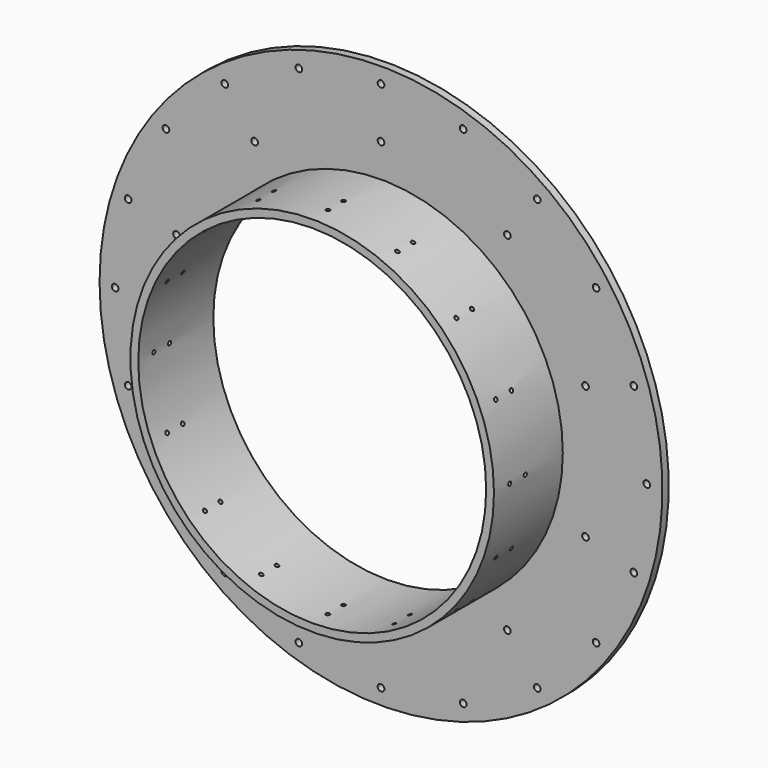
from build123d import *

# Parameters (mm, degrees)
F0_R            = 232.5
F0_R_2          = 222.5
F1_DEPTH        = 60
F2_R            = 360
F2_R_2          = 232.5
F3_DEPTH        = 10
F5_D            = 8.5
F5_DEPTH        = 30
F5_TIP          = 2.5536576309
F5_COPIES_COUNT = 10
F6_R            = 2.5
F7_DEPTH        = 300
F7_COPIES_COUNT = 16
F9_D            = 8.5
F9_DEPTH        = 22.1
F9_TIP          = 2.5536576309
F9_COPIES_COUNT = 20


# Not quite as in the source:
# - a pattern or mirror of a feature is missing from the dataset's text; its kind, count and spacing are read off the source's solid


with BuildPart() as f1:
    # F0 (on Front) → F1 (new body, symmetric)
    with BuildSketch(Plane.XZ):
        Circle(F0_R)
        Circle(F0_R_2, mode=Mode.SUBTRACT)
    extrude(amount=F1_DEPTH, both=True)

    # F2 (on face) → F3 (join)
    with BuildSketch(Plane(origin=(0, 60, 0), x_dir=(-1, 0, 0), z_dir=(0, 1, 0))):
        Circle(F2_R)
        Circle(F2_R_2, mode=Mode.SUBTRACT)
    extrude(amount=-F3_DEPTH)

    # F5
    with Locations(Plane(origin=(0, 60, 0), x_dir=(-1, 0, 0), z_dir=(0, 1, 0))):
        with Locations((0, 275)):
            f5 = Hole(F5_D / 2, depth=F5_DEPTH)
            with Locations((0, 0, -(F5_DEPTH + F5_TIP / 2))):  # 118° drill point
                Cone(0, F5_D / 2, F5_TIP, mode=Mode.SUBTRACT)

    # F5_copies: F5 ×10 about axis
    f5_copies_axis = Axis((0, 0, 0), (0, 1, 0))
    for i in range(1, F5_COPIES_COUNT):
        add(f5.rotate(f5_copies_axis, i * 360 / F5_COPIES_COUNT), mode=Mode.SUBTRACT)

    # F6 (on Top) → F7 (cut)
    with BuildSketch(Plane.XY):
        with Locations((0, -35)):
            Circle(F6_R)
        with Locations((0, -10)):
            Circle(F6_R)
    f7 = extrude(amount=F7_DEPTH, mode=Mode.SUBTRACT)

    # F7_copies: F7 ×16 about axis
    f7_copies_axis = Axis((0, 0, 0), (0, 1, 0))
    for i in range(1, F7_COPIES_COUNT):
        add(f7.rotate(f7_copies_axis, i * 360 / F7_COPIES_COUNT), mode=Mode.SUBTRACT)

    # F9
    with Locations(Plane(origin=(0, 60, 0), x_dir=(-1, 0, 0), z_dir=(0, 1, 0))):
        with Locations((0, 340)):
            f9 = Hole(F9_D / 2, depth=F9_DEPTH)
            with Locations((0, 0, -(F9_DEPTH + F9_TIP / 2))):  # 118° drill point
                Cone(0, F9_D / 2, F9_TIP, mode=Mode.SUBTRACT)

    # F9_copies: F9 ×20 about axis
    f9_copies_axis = Axis((0, 0, 0), (0, 1, 0))
    for i in range(1, F9_COPIES_COUNT):
        add(f9.rotate(f9_copies_axis, i * 360 / F9_COPIES_COUNT), mode=Mode.SUBTRACT)


solid = f1.part
